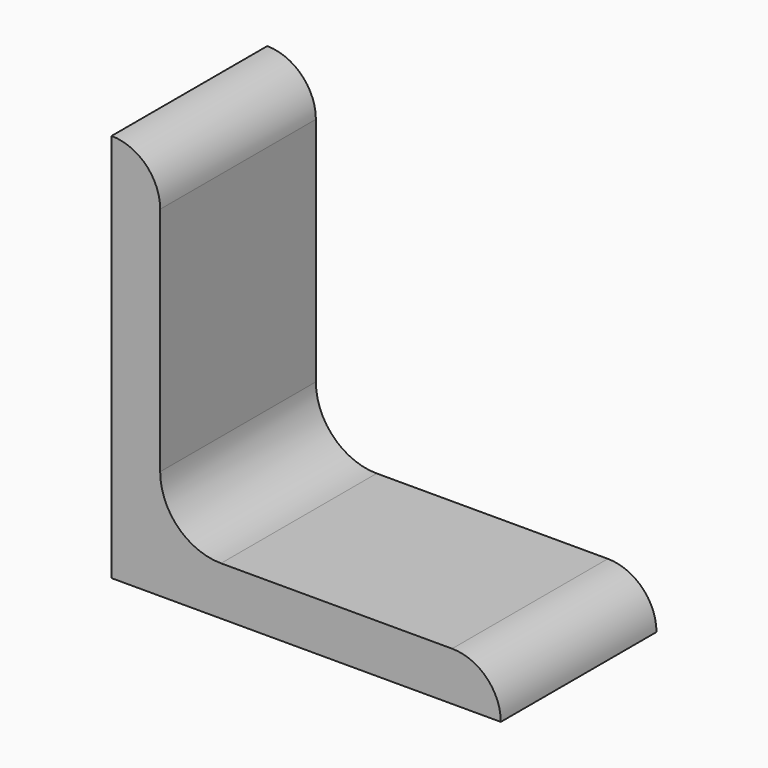
from build123d import *

# Parameters (mm, degrees)
F1_DEPTH = 12.7
F2_R     = 6.34999
F3_R     = 7.9375


# Not quite as in the source:
# - a fillet or chamfer is up to 0.001 mm smaller than in the source, because OpenCascade refuses the exact size


with BuildPart() as f1:
    # F0 (on Front) → F1 (new body, symmetric)
    with BuildSketch(Plane.XZ):
        Polygon((6.35, 50.8), (0, 50.8), (0, 0), (50.8, 0), (50.8, 6.35), (6.35, 6.35), align=None)
    extrude(amount=F1_DEPTH, both=True)

    # F2 (radius 6.35 in the source; OpenCascade refuses exactly that, so slightly less here)
    f2_edges = [f1.edges().sort_by_distance(p)[0] for p in [
        (6.35, 0, 50.8),
        (50.8, 0, 6.35),
    ]]
    fillet(f2_edges, radius=F2_R)

    # F3
    f3_edges = [f1.edges().sort_by_distance(p)[0] for p in [
        (6.35, 0, 6.35),
    ]]
    fillet(f3_edges, radius=F3_R)


solid = f1.part
